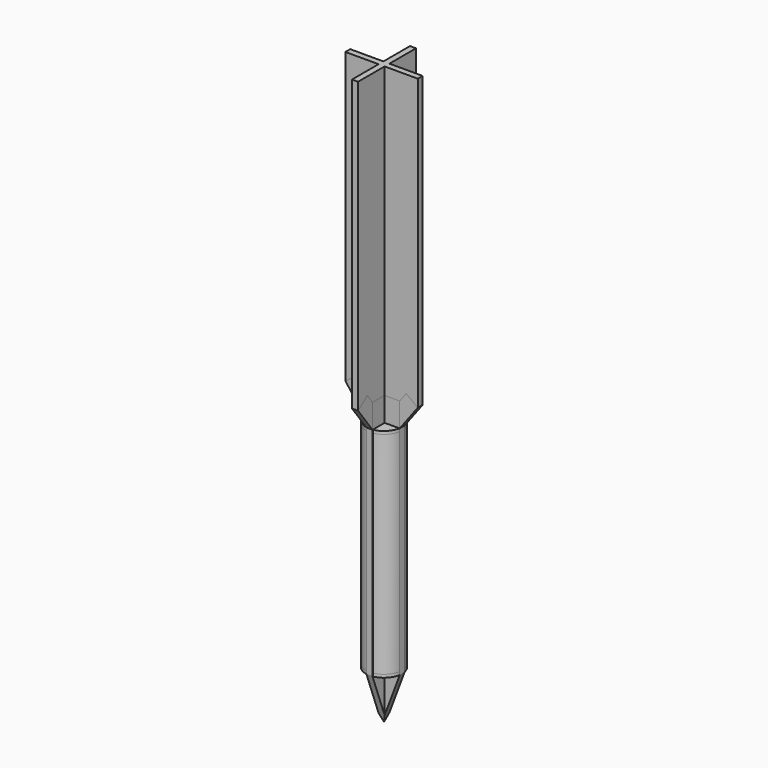
from build123d import *

# Parameters (mm, degrees)
F0_W           = 6.35
F0_H           = 34.925
F0_W_2         = 34.925
F0_H_2         = 6.35
F1_DEPTH       = 304.8
F2_W           = 15.875
F2_H           = 6.35
F2_W_2         = 6.35
F2_H_2         = 15.875
F3_DEPTH       = 254
F5_E4_W        = 31.7372608571
F5_E4_H        = 3.175
F6_DEPTH       = 15.24
F7_DEPTH       = 3.175
F9_E5_W        = 31.8220023402
F9_E5_H        = 3.175
F10_DEPTH      = 15.24
F11_DEPTH      = 3.175
F13_E6_W       = 31.75
F13_E6_H       = 3.175
F14_DEPTH      = 15.24
F15_DEPTH      = 3.175
F16_E7_W       = 31.75
F16_E7_H       = 3.175
F17_DEPTH      = 15.24
F18_DEPTH      = 3.175
F20_START      = -28.575
F19_R          = 19.05
F20_DEPTH      = 222.25
F22_START      = -25.4
F21_R          = 19.05
F22_DEPTH      = 3.175
F24_START      = -250.825
F23_R          = 19.05
F24_DEPTH      = 3.175
F26_DEPTH      = 3.175
F26_DEPTH_BACK = 3.175
F28_DEPTH      = 3.175
F28_DEPTH_BACK = 3.175
F30_DEPTH      = 25.4
F30_DEPTH_BACK = 25.4
F32_DEPTH      = 25.4
F32_DEPTH_BACK = 25.4
F34_DEPTH      = 25.4
F34_DEPTH_BACK = 25.4
F36_DEPTH      = 25.4
F36_DEPTH_BACK = 25.4


with BuildPart() as f1:
    # F0 (on Top) → F1 (new body)
    with BuildSketch(Plane.XY):
        with Locations((0, 20.6375)):
            Rectangle(F0_W, F0_H)
        with Locations((-20.6375, 0)):
            Rectangle(F0_W_2, F0_H_2)
        with Locations((0, -20.6375)):
            Rectangle(F0_W, F0_H)
        Rectangle(F0_W, F0_H_2)
        with Locations((20.6375, 0)):
            Rectangle(F0_W_2, F0_H_2)
    extrude(amount=F1_DEPTH)


with BuildPart() as f3:
    # F2 (on Top) → F3 (new body)
    with BuildSketch(Plane.XY):
        with Locations((11.1125, 0)):
            Rectangle(F2_W, F2_H)
        with Locations((-11.1125, 0)):
            Rectangle(F2_W, F2_H)
        with Locations((0, 11.1125)):
            Rectangle(F2_W_2, F2_H_2)
        with Locations((0, -11.1125)):
            Rectangle(F2_W_2, F2_H_2)
        Rectangle(F2_W_2, F2_H)
    extrude(amount=-F3_DEPTH)

    # F9_E5 (on explicit) → F10 (join)
    with BuildSketch(Plane(origin=(-38.1, 0, 0), x_dir=(0.6024059487, 0, -0.7981898728), z_dir=(-0.7981898728, 0, -0.6024059487))):
        with Locations((15.9110011701, 1.5875)):
            Rectangle(F9_E5_W, F9_E5_H)
    extrude(amount=-F10_DEPTH)


with BuildPart() as f6:
    # F5_E4 (on explicit) → F6 (new body)
    with BuildSketch(Plane(origin=(38.1, 0, 0), x_dir=(-0.5995716076, 0, -0.8003211151), z_dir=(-0.8003211151, 0, 0.5995716076))):
        with Locations((15.8686304286, 1.5875)):
            Rectangle(F5_E4_W, F5_E4_H)
    extrude(amount=F6_DEPTH)


with BuildPart() as f7:
    # F7 (new): a face of the model
    f7_faces = [f6.part.faces().sort_by_distance(p)[0] for p in [
        (22.4871728456, 0, -8.1312643497),
    ]]
    extrude(f7_faces, amount=F7_DEPTH)


with BuildPart() as f11:
    # F11 (new): a face of the model
    f11_faces = [f3.part.faces().sort_by_distance(p)[0] for p in [
        (-26.0093205112, 0, -5.3484628484),
    ]]
    extrude(f11_faces, amount=F11_DEPTH)


with BuildPart() as f14:
    # F13_E6 (on explicit) → F14 (new body)
    with BuildSketch(Plane(origin=(0, 38.1, 0), x_dir=(0, -0.6, -0.8), z_dir=(0, -0.8, 0.6))):
        with Locations((15.875, 1.5875)):
            Rectangle(F13_E6_W, F13_E6_H)
    extrude(amount=F14_DEPTH)


with BuildPart() as f15:
    # F15 (new): a face of the model
    f15_faces = [f14.part.faces().sort_by_distance(p)[0] for p in [
        (0, 22.479, -8.128),
    ]]
    extrude(f15_faces, amount=F15_DEPTH)


with BuildPart() as f17:
    # F16_E7 (on explicit) → F17 (new body)
    with BuildSketch(Plane(origin=(0, -38.1, 0), x_dir=(0, 0.6, -0.8), z_dir=(0, -0.8, -0.6))):
        with Locations((15.875, 1.5875)):
            Rectangle(F16_E7_W, F16_E7_H)
    extrude(amount=-F17_DEPTH)


with BuildPart() as f18:
    # F18 (new): a face of the model
    f18_faces = [f17.part.faces().sort_by_distance(p)[0] for p in [
        (0, -22.479, -8.128),
    ]]
    extrude(f18_faces, amount=F18_DEPTH)


with BuildPart() as f20:
    # F19 (on Top) → F20 (new body)
    with BuildSketch(Plane.XY.offset(F20_START)):
        Circle(F19_R)
    extrude(amount=-F20_DEPTH)


with BuildPart() as f22:
    # F21 (on Top) → F22 (new body)
    with BuildSketch(Plane.XY.offset(F22_START)):
        Circle(F21_R)
    extrude(amount=-F22_DEPTH)


with BuildPart() as f24:
    # F23 (on Top) → F24 (new body)
    with BuildSketch(Plane.XY.offset(F24_START)):
        Circle(F23_R)
    extrude(amount=-F24_DEPTH)


with BuildPart() as f3_1:
    add(f3.part)

    # F25 (on Front) → F26 (join, two sides)
    with BuildSketch(Plane.XZ) as f26_sk:
        Polygon((0, -304.8), (19.05, -254), (-19.05, -254), align=None)
    extrude(amount=F26_DEPTH)
    extrude(f26_sk.sketch, amount=-F26_DEPTH_BACK)

    # F27 (on Right) → F28 (join, two sides)
    with BuildSketch(Plane.YZ) as f28_sk:
        Polygon((19.05, -253.961299397), (-19.05, -254), (0, -304.8), align=None)
    extrude(amount=F28_DEPTH)
    extrude(f28_sk.sketch, amount=-F28_DEPTH_BACK)

    # F29 (on Front) → F30 (cut, two sides)
    with BuildSketch(Plane.XZ) as f30_sk:
        Polygon((14.5053900778, -306.9541752338), (19.05, -254), (0, -304.8), align=None)
    extrude(amount=-F30_DEPTH, mode=Mode.SUBTRACT)
    extrude(f30_sk.sketch, amount=F30_DEPTH_BACK, mode=Mode.SUBTRACT)

    # F31 (on Front) → F32 (cut, two sides)
    with BuildSketch(Plane.XZ) as f32_sk:
        Polygon((0, -304.8), (-19.05, -254), (-17.9964636892, -308.1513562202), align=None)
    extrude(amount=-F32_DEPTH, mode=Mode.SUBTRACT)
    extrude(f32_sk.sketch, amount=F32_DEPTH_BACK, mode=Mode.SUBTRACT)

    # F33 (on Right) → F34 (cut, two sides)
    with BuildSketch(Plane.YZ) as f34_sk:
        Polygon((0, -304.8), (-19.0134039452, -254.0975894796), (-19.4287896156, -254.4830143452), (-21.6469541192, -304.8), align=None)
    extrude(amount=-F34_DEPTH, mode=Mode.SUBTRACT)
    extrude(f34_sk.sketch, amount=F34_DEPTH_BACK, mode=Mode.SUBTRACT)

    # F35 (on Right) → F36 (cut, two sides)
    with BuildSketch(Plane.YZ) as f36_sk:
        Polygon((28.5147875547, -304.8), (19.05, -254), (0, -304.8), align=None)
    extrude(amount=-F36_DEPTH, mode=Mode.SUBTRACT)
    extrude(f36_sk.sketch, amount=F36_DEPTH_BACK, mode=Mode.SUBTRACT)


solid = Compound([f1.part, f6.part, f7.part, f11.part, f14.part, f15.part, f17.part, f18.part, f20.part, f22.part, f24.part, f3_1.part])
